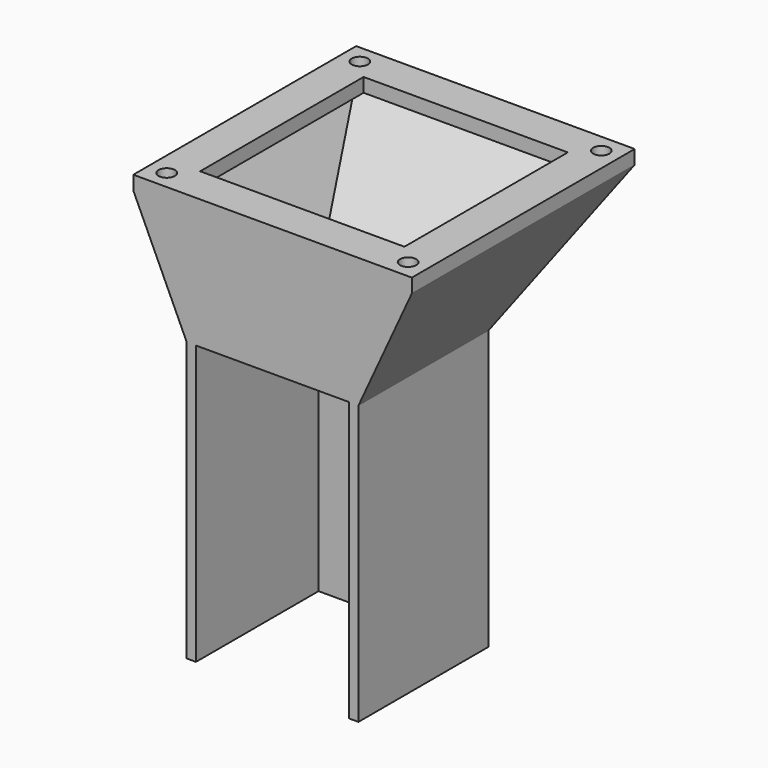
from build123d import *

# Parameters (mm, degrees)
F1_DEPTH = 60
F3_R     = 1.75
F3_W     = 3.5
F3_H     = 8
F3_W_2   = 2
F3_W_3   = 33
F4_DEPTH = 3
F6_W     = 37
F6_H     = 35
F5_W     = 60
F5_H     = 60
F10_W    = 56
F10_H    = 56


# Not quite as in the source:
# - a feature names something its author has since deleted; it is built from what else it names


with BuildPart() as f1:
    # F0 (on Top) → F1 (new body)
    with BuildSketch(Plane.XY):
        Polygon((-2, 0), (0, 0), (0, 33), (33, 33), (33, 0), (35, 0), (35, 35), (-2, 35), align=None)
    extrude(amount=F1_DEPTH)



with BuildPart() as f4:
    # F3 (on offset) → F4 (new body)
    with BuildSketch(Plane.XY.offset(85)):
        Polygon((-13.5, 0), (-5.5, 0), (-5.5, 8), (-5.5, 52), (38.5, 52), (38.5, 8), (38.5, 0), (46.5, 0), (46.5, 60), (-13.5, 60), align=None)
        with Locations((-9.5, 4)):
            Circle(F3_R, mode=Mode.SUBTRACT)
        with Locations((42.5, 4)):
            Circle(F3_R, mode=Mode.SUBTRACT)
        with Locations((-9.5, 56)):
            Circle(F3_R, mode=Mode.SUBTRACT)
        with Locations((42.5, 56)):
            Circle(F3_R, mode=Mode.SUBTRACT)
        with Locations((-3.75, 4)):
            Rectangle(F3_W, F3_H)
        with Locations((36.75, 4)):
            Rectangle(F3_W, F3_H)
        with Locations((34, 4)):
            Rectangle(F3_W_2, F3_H)
        with Locations((-1, 4)):
            Rectangle(F3_W_2, F3_H)
        with Locations((16.5, 4)):
            Rectangle(F3_W_3, F3_H)
    extrude(amount=F4_DEPTH)


with BuildPart() as f1_1:
    add(f1.part)

    add(f4.part)  # F7 merges F4
    # F6 (on face) → F7 section 0
    with BuildSketch(Plane.XY.offset(60)):
        with Locations((16.5, 17.5)):
            Rectangle(F6_W, F6_H)
    # F5 (on face) → F7 section 1
    with BuildSketch(Plane.XY.offset(85)):
        with Locations((16.5, 30)):
            Rectangle(F5_W, F5_H)
    loft()


with BuildPart() as f11:
    # F10 (on offset) → F11 section 0
    with BuildSketch(Plane(origin=(0, 0, 85), x_dir=(1, 0, 0), z_dir=(0, 0, -1))):
        with Locations((16.5, -30)):
            Rectangle(F10_W, F10_H)
    # F9 (on face) → F11 section 1
    with BuildSketch(Plane.XY.offset(60)):
        Polygon((0, 33), (0, 2), (2, 2), (4, 2), (29, 2), (31, 2), (33, 2), (33, 33), align=None)
    loft()


with BuildPart() as f1_2:
    add(f1_1.part)

    # F13: cut F11
    add(f11.part, mode=Mode.SUBTRACT)


solid = f1_2.part
